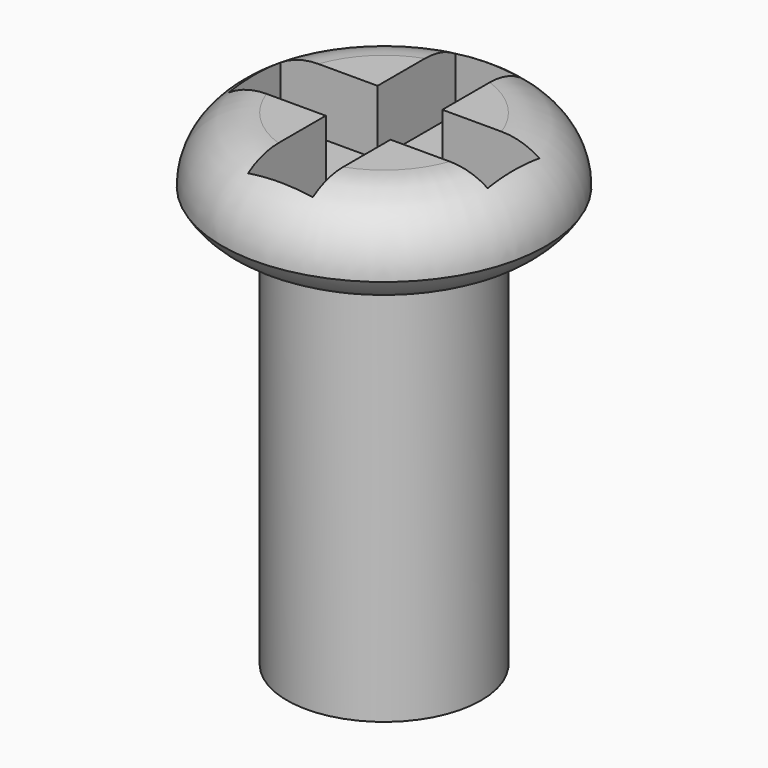
from build123d import *

# Parameters (mm, degrees)
F0_R     = 1.5
F1_DEPTH = 6
F2_R     = 2.5
F3_DEPTH = 1.5
F4_W     = 1
F4_H     = 1.5
F4_H_2   = 1
F4_W_2   = 1.5
F5_DEPTH = 1


# Not quite as in the source:
# - a fillet or chamfer that OpenCascade refuses, or shapes differently, is made with other operations: its cross-section is extruded or revolved along the edge and cut away or added


with BuildPart() as f1:
    # F0 (on Top) → F1 (new body)
    with BuildSketch(Plane.XY):
        Circle(F0_R)
    extrude(amount=F1_DEPTH)

    # F2 (on face) → F3 (join)
    with BuildSketch(Plane.XY.offset(6)):
        Circle(F2_R)
    extrude(amount=F3_DEPTH)

    # F4 (on face) → F5 (cut)
    with BuildSketch(Plane.XY.offset(7.5)):
        with Locations((0, 1.25)):
            Rectangle(F4_W, F4_H)
        Rectangle(F4_W, F4_H_2)
        with Locations((-1.25, 0)):
            Rectangle(F4_W_2, F4_H_2)
        with Locations((1.25, 0)):
            Rectangle(F4_W_2, F4_H_2)
        with Locations((0, -1.25)):
            Rectangle(F4_W, F4_H)
    extrude(amount=-F5_DEPTH, mode=Mode.SUBTRACT)

    # F6: fillet of radius 1 on 1 edges, made by hand

    # F6_s1 → F6_t2 (revolve, cut)
    with BuildSketch(Plane.XZ):
        with BuildLine():
            ThreePointArc((2.5, 6.5), (2.2071067812, 7.2071067812), (1.5, 7.5))
            Line((1.5, 7.5), (2.5, 7.5))
            Line((2.5, 7.5), (2.5, 6.5))
        make_face()
    revolve(axis=Axis((0, 0, 7.5), (0, 0, 1)), mode=Mode.SUBTRACT)

    # F7: fillet of radius 1 on 1 edges, made by hand

    # F7_s1 → F7_t2 (revolve, cut)
    with BuildSketch(Plane.XZ):
        with BuildLine():
            ThreePointArc((2.5, 6.5), (2.1339745962, 6.1339745962), (1.6339745962, 6))
            Line((1.6339745962, 6), (2.5, 6))
            Line((2.5, 6), (2.5, 6.5))
        make_face()
    revolve(axis=Axis((0, 0, 6), (0, 0, 1)), mode=Mode.SUBTRACT)


solid = f1.part
